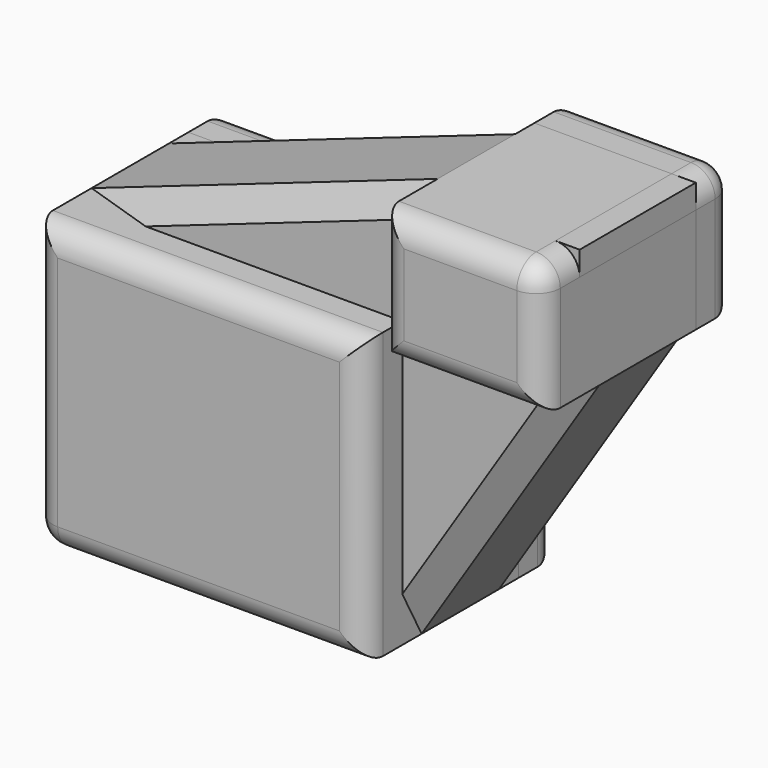
from build123d import *

# Parameters (mm, degrees)
F0_W           = 68.229958415
F0_H           = 58.9122157544
F1_DEPTH       = 40
F0_W_2         = 33.3635509014
F0_H_2         = 26.750953868
F2_DEPTH       = 30
F3_R           = 5
F4_SIZE        = 5
F5_DEPTH       = 10
F6_T1_DEPTH    = 47.5
F6_S5_W        = 5
F6_S5_H        = 5
F6_T6_DEPTH    = 5
F6_2_T1_DEPTH  = 51.750953868
F6_2_T3_DEPTH  = 34.250953868
F6_2_T5_DEPTH  = 58.3635509014
F6_2_T7_DEPTH  = 40.8635509014
F6_2_T9_DEPTH  = 47.5
F6_2_S13_W     = 5
F6_2_S13_H     = 5
F6_2_T14_DEPTH = 5
F6_3_T1_DEPTH  = 55
F6_4_T1_DEPTH  = 93.229958415
F6_4_T3_DEPTH  = 83.9122157544
F6_4_T5_DEPTH  = 66.4122157544
F6_4_T7_DEPTH  = 75.729958415
F6_4_T9_DEPTH  = 17.5
F6_4_S13_W     = 5
F6_4_S13_H     = 5
F6_4_T14_DEPTH = 5
F6_5_T1_DEPTH  = 40.8635509014
F6_5_T3_DEPTH  = 34.250953868
F6_5_T5_DEPTH  = 58.3635509014
F6_5_T7_DEPTH  = 51.750953868
F6_5_T9_DEPTH  = 17.5
F6_5_S13_W     = 5
F6_5_S13_H     = 5
F6_5_T14_DEPTH = 5


# Not quite as in the source:
# - a fillet or chamfer that OpenCascade refuses, or shapes differently, is made with other operations: its cross-section is extruded or revolved along the edge and cut away or added


with BuildPart() as f1:
    # F0 (on Front) → F1 (new body)
    with BuildSketch(Plane.XZ):
        with Locations((-0.6011463702, -2.2542933002)):
            Rectangle(F0_W, F0_H)
    extrude(amount=F1_DEPTH)

    # F3
    f3_edges = [f1.edges().sort_by_distance(p)[0] for p in [
        (-0.601146, -40, 27.201815),
        (-34.716126, -40, -2.254293),
        (-0.601146, -40, -31.710401),
        (33.513833, -40, -2.254293),
    ]]
    fillet(f3_edges, radius=F3_R)


with BuildPart() as f1b:
    # F0 (on Front) → F1, piece 2 (new body)
    with BuildSketch(Plane.XZ):
        with Locations((53.5019114614, 38.7738561258)):
            Rectangle(F0_W_2, F0_H_2)
    extrude(amount=F1_DEPTH)


with BuildPart() as f2:
    # F0 (on Front) → F2 (new body)
    with BuildSketch(Plane.XZ):
        Polygon((36.8201360106, 52.1493330598), (-34.7161255777, 27.201814577), (33.5138328373, 27.201814577), (33.5138328373, -31.7104011774), (70.1836869121, 25.3983791918), (36.8201360106, 25.3983791918), align=None)
        with Locations((-0.6011463702, -2.2542933002)):
            Rectangle(F0_W, F0_H)
        with Locations((53.5019114614, 38.7738561258)):
            Rectangle(F0_W_2, F0_H_2)
    extrude(amount=F2_DEPTH)

    # F4
    f4_edges = [f2.edges().sort_by_distance(p)[0] for p in [
        (1.052005, -30, 39.675574),
        (1.052005, 0, 39.675574),
        (51.84876, -30, -3.156011),
        (51.84876, 0, -3.156011),
    ]]
    chamfer(f4_edges, length=F4_SIZE)

    # F6#3: fillet of radius 5 on 1 edges, made by hand

    # F6_3_s2 → F6_3_t1 (cut)
    with BuildSketch(Plane.XZ.offset(-12.5)):
        with BuildLine():
            ThreePointArc((-34.7161255777, -26.7104011774), (-33.2516594836, -30.2459350833), (-29.7161255777, -31.7104011774))
            Line((-29.7161255777, -31.7104011774), (-34.7161255777, -31.7104011774))
            Line((-34.7161255777, -31.7104011774), (-34.7161255777, -26.7104011774))
        make_face()
    extrude(amount=F6_3_T1_DEPTH, mode=Mode.SUBTRACT)


with BuildPart() as f5:
    # F5 (new): a face of the model
    f5_faces = [f1.part.faces().sort_by_distance(p)[0] for p in [
        (-0.6011463702, 0, -2.2542933002),
    ]]
    extrude(f5_faces, amount=F5_DEPTH)

    # F6#4: fillet of radius 5 on 5 edges, made by hand

    # F6_4_s2 → F6_4_t1 (cut)
    with BuildSketch(Plane.YZ.offset(-47.2161255777)):
        with BuildLine():
            ThreePointArc((5, 27.201814577), (8.5355339059, 25.7373484829), (10, 22.201814577))
            Line((10, 22.201814577), (10, 27.201814577))
            Line((10, 27.201814577), (5, 27.201814577))
        make_face()
    extrude(amount=F6_4_T1_DEPTH, mode=Mode.SUBTRACT)

    # F6_4_s4 → F6_4_t3 (cut)
    with BuildSketch(Plane.XY.offset(-44.2104011774)):
        with BuildLine():
            ThreePointArc((33.5138328373, 5), (32.0493667433, 8.5355339059), (28.5138328373, 10))
            Line((28.5138328373, 10), (33.5138328373, 10))
            Line((33.5138328373, 10), (33.5138328373, 5))
        make_face()
    extrude(amount=F6_4_T3_DEPTH, mode=Mode.SUBTRACT)

    # F6_4_s6 → F6_4_t5 (cut)
    with BuildSketch(Plane.XY.offset(-26.7104011774)):
        with BuildLine():
            ThreePointArc((-34.7161255777, 5), (-33.2516594836, 8.5355339059), (-29.7161255777, 10))
            Line((-29.7161255777, 10), (-34.7161255777, 10))
            Line((-34.7161255777, 10), (-34.7161255777, 5))
        make_face()
    extrude(amount=F6_4_T5_DEPTH, mode=Mode.SUBTRACT)

    # F6_4_s8 → F6_4_t7 (cut)
    with BuildSketch(Plane.YZ.offset(-29.7161255777)):
        with BuildLine():
            ThreePointArc((5, -31.7104011774), (8.5355339059, -30.2459350833), (10, -26.7104011774))
            Line((10, -26.7104011774), (10, -31.7104011774))
            Line((10, -31.7104011774), (5, -31.7104011774))
        make_face()
    extrude(amount=F6_4_T7_DEPTH, mode=Mode.SUBTRACT)

    # F6_4_s10 → F6_4_t9 (cut)
    with BuildSketch(Plane.XZ.offset(-5)):
        with BuildLine():
            ThreePointArc((-34.7161255777, -26.7104011774), (-33.2516594836, -30.2459350833), (-29.7161255777, -31.7104011774))
            Line((-29.7161255777, -31.7104011774), (-34.7161255777, -31.7104011774))
            Line((-34.7161255777, -31.7104011774), (-34.7161255777, -26.7104011774))
        make_face()
    extrude(amount=F6_4_T9_DEPTH, mode=Mode.SUBTRACT)


with BuildPart() as f5b:
    # F5#2 (new): a face of the model
    f5_2_faces = [f1b.part.faces().sort_by_distance(p)[0] for p in [
        (53.5019114614, 0, 38.7738561258),
    ]]
    extrude(f5_2_faces, amount=F5_DEPTH)

    # F6#5: fillet of radius 5 on 5 edges, made by hand

    # F6_5_s2 → F6_5_t1 (cut)
    with BuildSketch(Plane.YZ.offset(24.3201360106)):
        with BuildLine():
            ThreePointArc((5, 52.1493330598), (8.5355339059, 50.6848669657), (10, 47.1493330598))
            Line((10, 47.1493330598), (10, 52.1493330598))
            Line((10, 52.1493330598), (5, 52.1493330598))
        make_face()
    extrude(amount=F6_5_T1_DEPTH, mode=Mode.SUBTRACT)

    # F6_5_s4 → F6_5_t3 (cut)
    with BuildSketch(Plane.XY.offset(12.8983791918)):
        with BuildLine():
            ThreePointArc((70.1836869121, 5), (68.719220818, 8.5355339059), (65.1836869121, 10))
            Line((65.1836869121, 10), (70.1836869121, 10))
            Line((70.1836869121, 10), (70.1836869121, 5))
        make_face()
    extrude(amount=F6_5_T3_DEPTH, mode=Mode.SUBTRACT)

    # F6_5_s6 → F6_5_t5 (cut)
    with BuildSketch(Plane.YZ.offset(24.3201360106)):
        with BuildLine():
            ThreePointArc((5, 25.3983791918), (8.5355339059, 26.8628452858), (10, 30.3983791918))
            Line((10, 30.3983791918), (10, 25.3983791918))
            Line((10, 25.3983791918), (5, 25.3983791918))
        make_face()
    extrude(amount=F6_5_T5_DEPTH, mode=Mode.SUBTRACT)

    # F6_5_s8 → F6_5_t7 (cut)
    with BuildSketch(Plane.XY.offset(12.8983791918)):
        with BuildLine():
            ThreePointArc((36.8201360106, 5), (38.2846021047, 8.5355339059), (41.8201360106, 10))
            Line((41.8201360106, 10), (36.8201360106, 10))
            Line((36.8201360106, 10), (36.8201360106, 5))
        make_face()
    extrude(amount=F6_5_T7_DEPTH, mode=Mode.SUBTRACT)

    # F6_5_s10 → F6_5_t9 (cut)
    with BuildSketch(Plane.XZ.offset(-5)):
        with BuildLine():
            ThreePointArc((65.1836869121, 52.1493330598), (68.719220818, 50.6848669657), (70.1836869121, 47.1493330598))
            Line((70.1836869121, 47.1493330598), (70.1836869121, 52.1493330598))
            Line((70.1836869121, 52.1493330598), (65.1836869121, 52.1493330598))
        make_face()
    extrude(amount=F6_5_T9_DEPTH, mode=Mode.SUBTRACT)


with BuildPart() as f1_1:
    add(f1.part)

    # F6: fillet of radius 5 on 1 edges, made by hand

    # F6_s2 → F6_t1 (cut)
    with BuildSketch(Plane.XZ.offset(-12.5)):
        with BuildLine():
            ThreePointArc((-34.7161255777, -26.7104011774), (-33.2516594836, -30.2459350833), (-29.7161255777, -31.7104011774))
            Line((-29.7161255777, -31.7104011774), (-34.7161255777, -31.7104011774))
            Line((-34.7161255777, -31.7104011774), (-34.7161255777, -26.7104011774))
        make_face()
    extrude(amount=F6_T1_DEPTH, mode=Mode.SUBTRACT)


with BuildPart() as f6_tool4:
    # F6_s5 → F6_t6 (new body)
    with BuildSketch(Plane.YZ.offset(-29.7161255777)):
        with Locations((-37.5, -29.2104011774)):
            Rectangle(F6_S5_W, F6_S5_H)
    extrude(amount=-F6_T6_DEPTH)

    # F6_s7 → F6_t8 (revolve, cut)
    with BuildSketch(Plane(origin=(-29.7161255777, -35, -26.7104011774), x_dir=(0, 0.7071067812, 0.7071067812), z_dir=(0, -0.7071067812, 0.7071067812))):
        with BuildLine():
            ThreePointArc((0, -5), (5, 0), (0, 5))
            Line((0, 5), (0, -5))
        make_face()
    revolve(axis=Axis((-29.7161255777, -35, -26.7104011774), (-1, 0, 0)), mode=Mode.SUBTRACT)


with BuildPart() as f1_2:
    add(f1_1.part)

    # F6_t3: cut F6_tool4
    add(f6_tool4.part, mode=Mode.SUBTRACT)


with BuildPart() as f1b_1:
    add(f1b.part)

    # F6#2: fillet of radius 5 on 5 edges, made by hand

    # F6_2_s2 → F6_2_t1 (cut)
    with BuildSketch(Plane.XY.offset(12.8983791918)):
        with BuildLine():
            ThreePointArc((36.8201360106, -35), (38.2846021047, -38.5355339059), (41.8201360106, -40))
            Line((41.8201360106, -40), (36.8201360106, -40))
            Line((36.8201360106, -40), (36.8201360106, -35))
        make_face()
    extrude(amount=F6_2_T1_DEPTH, mode=Mode.SUBTRACT)

    # F6_2_s4 → F6_2_t3 (cut)
    with BuildSketch(Plane.XY.offset(12.8983791918)):
        with BuildLine():
            ThreePointArc((70.1836869121, -35), (68.719220818, -38.5355339059), (65.1836869121, -40))
            Line((65.1836869121, -40), (70.1836869121, -40))
            Line((70.1836869121, -40), (70.1836869121, -35))
        make_face()
    extrude(amount=F6_2_T3_DEPTH, mode=Mode.SUBTRACT)

    # F6_2_s6 → F6_2_t5 (cut)
    with BuildSketch(Plane.YZ.offset(24.3201360106)):
        with BuildLine():
            ThreePointArc((-35, 25.3983791918), (-38.5355339059, 26.8628452858), (-40, 30.3983791918))
            Line((-40, 30.3983791918), (-40, 25.3983791918))
            Line((-40, 25.3983791918), (-35, 25.3983791918))
        make_face()
    extrude(amount=F6_2_T5_DEPTH, mode=Mode.SUBTRACT)

    # F6_2_s8 → F6_2_t7 (cut)
    with BuildSketch(Plane.YZ.offset(24.3201360106)):
        with BuildLine():
            ThreePointArc((-35, 52.1493330598), (-38.5355339059, 50.6848669657), (-40, 47.1493330598))
            Line((-40, 47.1493330598), (-40, 52.1493330598))
            Line((-40, 52.1493330598), (-35, 52.1493330598))
        make_face()
    extrude(amount=F6_2_T7_DEPTH, mode=Mode.SUBTRACT)

    # F6_2_s10 → F6_2_t9 (cut)
    with BuildSketch(Plane.XZ.offset(-12.5)):
        with BuildLine():
            ThreePointArc((65.1836869121, 52.1493330598), (68.719220818, 50.6848669657), (70.1836869121, 47.1493330598))
            Line((70.1836869121, 47.1493330598), (70.1836869121, 52.1493330598))
            Line((70.1836869121, 52.1493330598), (65.1836869121, 52.1493330598))
        make_face()
    extrude(amount=F6_2_T9_DEPTH, mode=Mode.SUBTRACT)


with BuildPart() as f6_2_tool12:
    # F6_2_s13 → F6_2_t14 (new body)
    with BuildSketch(Plane.XY.offset(47.1493330598)):
        with Locations((67.6836869121, -37.5)):
            Rectangle(F6_2_S13_W, F6_2_S13_H)
    extrude(amount=F6_2_T14_DEPTH)

    # F6_2_s15 → F6_2_t16 (revolve, cut)
    with BuildSketch(Plane(origin=(65.1836869121, -35, 47.1493330598), x_dir=(-0.7071067812, 0.7071067812, 0), z_dir=(0.7071067812, 0.7071067812, 0))):
        with BuildLine():
            ThreePointArc((0, -5), (5, 0), (0, 5))
            Line((0, 5), (0, -5))
        make_face()
    revolve(axis=Axis((65.1836869121, -35, 47.1493330598), (0, 0, 1)), mode=Mode.SUBTRACT)


with BuildPart() as f1b_2:
    add(f1b_1.part)

    # F6_2_t11: cut F6_2_tool12
    add(f6_2_tool12.part, mode=Mode.SUBTRACT)


with BuildPart() as f6_4_tool12:
    # F6_4_s13 → F6_4_t14 (new body)
    with BuildSketch(Plane.YZ.offset(-29.7161255777)):
        with Locations((7.5, -29.2104011774)):
            Rectangle(F6_4_S13_W, F6_4_S13_H)
    extrude(amount=-F6_4_T14_DEPTH)

    # F6_4_s15 → F6_4_t16 (revolve, cut)
    with BuildSketch(Plane(origin=(-29.7161255777, 5, -26.7104011774), x_dir=(0, -0.7071067812, 0.7071067812), z_dir=(0, -0.7071067812, -0.7071067812))):
        with BuildLine():
            ThreePointArc((0, -5), (5, 0), (0, 5))
            Line((0, 5), (0, -5))
        make_face()
    revolve(axis=Axis((-29.7161255777, 5, -26.7104011774), (-1, 0, 0)), mode=Mode.SUBTRACT)


with BuildPart() as f5_1:
    add(f5.part)

    # F6_4_t11: cut F6_4_tool12
    add(f6_4_tool12.part, mode=Mode.SUBTRACT)


with BuildPart() as f6_5_tool12:
    # F6_5_s13 → F6_5_t14 (new body)
    with BuildSketch(Plane.XY.offset(47.1493330598)):
        with Locations((67.6836869121, 7.5)):
            Rectangle(F6_5_S13_W, F6_5_S13_H)
    extrude(amount=F6_5_T14_DEPTH)

    # F6_5_s15 → F6_5_t16 (revolve, cut)
    with BuildSketch(Plane(origin=(65.1836869121, 5, 47.1493330598), x_dir=(-0.7071067812, -0.7071067812, 0), z_dir=(-0.7071067812, 0.7071067812, 0))):
        with BuildLine():
            ThreePointArc((0, -5), (5, 0), (0, 5))
            Line((0, 5), (0, -5))
        make_face()
    revolve(axis=Axis((65.1836869121, 5, 47.1493330598), (0, 0, 1)), mode=Mode.SUBTRACT)


with BuildPart() as f5b_1:
    add(f5b.part)

    # F6_5_t11: cut F6_5_tool12
    add(f6_5_tool12.part, mode=Mode.SUBTRACT)


solid = Compound([f2.part, f1_2.part, f1b_2.part, f5_1.part, f5b_1.part])
